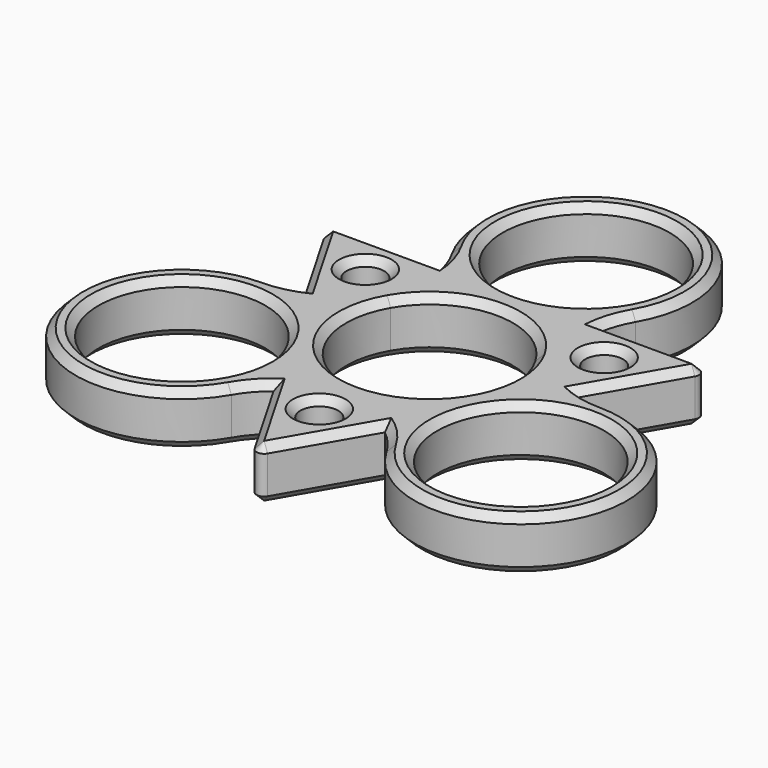
from build123d import *

# Parameters (mm, degrees)
F0_R            = 11.1
F1_DEPTH        = 7
F2_COUNT        = 3
F5_DEPTH        = 7
F5_COPIES_COUNT = 3
F6_D            = 5
F6_COPIES_COUNT = 3
F7_R            = 1
F8_SIZE         = 0.99999


# Not quite as in the source:
# - a fillet or chamfer is up to 0.001 mm smaller than in the source, because OpenCascade refuses the exact size
# - a pattern or mirror of a feature is missing from the dataset's text; its kind, count and spacing are read off the source's solid


with BuildPart() as f1:
    # F0 (on Top) → F1 (new body)
    with BuildSketch(Plane.XY):
        with BuildLine():
            ThreePointArc((-9.612881982, 5.55), (0, 11.1), (9.612881982, 5.55))
            Line((9.612881982, 5.55), (11.2583302492, 6.5))
            Line((11.2583302492, 6.5), (12.2109581934, 7.05))
            ThreePointArc((12.2109581934, 7.05), (10.6166604984, 13), (12.2109581934, 18.95))
            ThreePointArc((12.2109581934, 18.95), (0, 40.1), (-12.2109581934, 18.95))
            ThreePointArc((-12.2109581934, 18.95), (-10.6166604984, 13), (-12.2109581934, 7.05))
            Line((-12.2109581934, 7.05), (-11.2583302492, 6.5))
            Line((-11.2583302492, 6.5), (-9.612881982, 5.55))
        make_face()
        with Locations((0, 26)):
            Circle(F0_R, mode=Mode.SUBTRACT)
    extrude(amount=F1_DEPTH)

    # F2: F1 ×3 about axis
    f2_axis = Axis((0, 0, 0), (0, 0, 1))


with BuildPart() as f1_1:
    add(f1.part)
    for i in range(1, F2_COUNT):
        add(f1.part.rotate(f2_axis, i * 360 / F2_COUNT))

    # F4 (on face) → F5 (join)
    with BuildSketch(Plane.XY.offset(7)):
        with BuildLine():
            ThreePointArc((-18.1411493779, 1.9336138494), (-12.2109581934, 7.05), (-10.7451334036, 14.7438892904))
            Line((-10.7451334036, 14.7438892904), (-25.5371653521, 14.7438892904))
            Line((-25.5371653521, 14.7438892904), (-18.1411493779, 1.9336138494))
        make_face()
    f5 = extrude(amount=-F5_DEPTH)

    # F5_copies: F5 ×3 about axis
    f5_copies_axis = Axis((0, 0, 0), (0, 0, 1))
    for i in range(1, F5_COPIES_COUNT):
        add(f5.rotate(f5_copies_axis, i * 360 / F5_COPIES_COUNT))

    # F6 (through all)
    with Locations(Plane.XY.offset(7)):
        with Locations((-15.8686004579, 9.161740746)):
            f6 = Hole(F6_D / 2)

    # F6_copies: F6 ×3 about axis
    f6_copies_axis = Axis((0, 0, 0), (0, 0, 1))
    for i in range(1, F6_COPIES_COUNT):
        add(f6.rotate(f6_copies_axis, i * 360 / F6_COPIES_COUNT), mode=Mode.SUBTRACT)

    # F7
    f7_edges = [f1_1.edges().sort_by_distance(p)[0] for p in [
        (-25.537165, 14.743889, 3.5),
        (25.537165, 14.743889, 3.5),
        (0, -29.487779, 3.5),
    ]]
    fillet(f7_edges, radius=F7_R)

    # F8 (size 1 in the source; OpenCascade refuses exactly that, so slightly less here)
    f8_edges = [f1_1.edges().sort_by_distance(p)[0] for p in [
        (17.275124, 14.743889, 0),
        (24.67114, 14.243889, 0),
        (11.279496, 16.916139, 0),
        (21.406145, 7.588752, 0),
        (0, 40.1, 0),
        (20.289554, 1.310261, 0),
        (-11.279496, 16.916139, 0),
        (34.727619, -20.05, 0),
        (-17.275124, 14.743889, 0),
        (9.010058, -18.2264, 0),
        (-24.67114, 14.243889, 0),
        (4.131021, -22.332641, 0),
        (-21.406145, 7.588752, 0),
        (0, -28.487779, 0),
        (-20.289554, 1.310261, 0),
        (-4.131021, -22.332641, 0),
        (-34.727619, -20.05, 0),
        (-9.010058, -18.2264, 0),
        (-16.96666, -22.612882, 0),
        (1.25, -20.488545, 0),
        (28.06666, -3.387118, 0),
        (-9.612882, -5.55, 0),
        (-18.3686, 9.161741, 0),
        (17.1186, 11.326804, 0),
        (-11.1, 26, 0),
        (17.275124, 14.743889, 7),
        (24.67114, 14.243889, 7),
        (11.279496, 16.916139, 7),
        (21.406145, 7.588752, 7),
        (0, 40.1, 7),
        (20.289554, 1.310261, 7),
        (-11.279496, 16.916139, 7),
        (34.727619, -20.05, 7),
        (-17.275124, 14.743889, 7),
        (9.010058, -18.2264, 7),
        (-24.67114, 14.243889, 7),
        (4.131021, -22.332641, 7),
        (-21.406145, 7.588752, 7),
        (0, -28.487779, 7),
        (-20.289554, 1.310261, 7),
        (-4.131021, -22.332641, 7),
        (-34.727619, -20.05, 7),
        (-9.010058, -18.2264, 7),
        (-16.96666, -22.612882, 7),
        (1.25, -20.488545, 7),
        (28.06666, -3.387118, 7),
        (-9.612882, -5.55, 7),
        (-18.3686, 9.161741, 7),
        (17.1186, 11.326804, 7),
        (-11.1, 26, 7),
    ]]
    chamfer(f8_edges, length=F8_SIZE)


solid = f1_1.part
